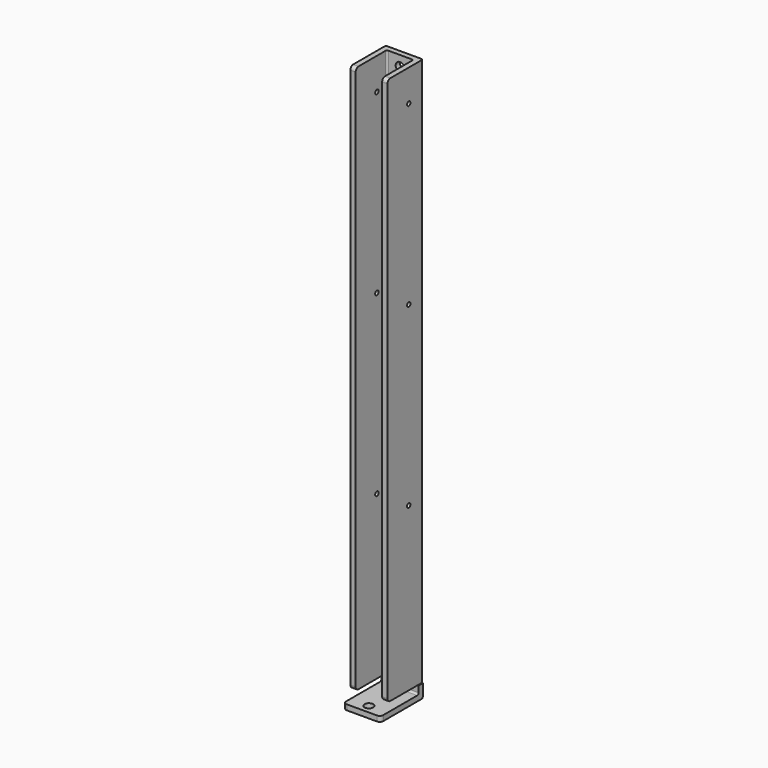
from build123d import *

# Parameters (mm, degrees)
F1_DEPTH  = 15
F2_W      = 3
F2_H      = 310
F3_DEPTH  = 25
F4_R      = 2.5
F5_DEPTH  = 3
F6_W      = 1
F6_H      = 0.5
F7_DEPTH  = 3
F8_R      = 1
F9_R      = 2.5
F9_R_2    = 1.2
F10_DEPTH = 3
F11_R     = 1.2
F12_DEPTH = 34.2
F13_DEPTH = 3
F14_DEPTH = 3
F15_R     = 2


with BuildPart() as f1:
    # F0 (on Right) → F1 (new body)
    with BuildSketch(Plane.YZ):
        Polygon((-7.5968508422, 3), (-7.5968508422, 0), (22.4031491578, 0), (22.4031491578, 318), (19.4031491578, 318), (19.4031491578, 3), align=None)
    extrude(amount=F1_DEPTH)

    # F2 (on face) → F3 (join)
    with BuildSketch(Plane(origin=(0, 22.4031491578, 0), x_dir=(-1, 0, 0), z_dir=(0, 1, 0))):
        with Locations((1.5, 163)):
            Rectangle(F2_W, F2_H)
        with Locations((-16.5, 163)):
            Rectangle(F2_W, F2_H)
    extrude(amount=-F3_DEPTH)

    # F4 (on face) → F5 (cut)
    with BuildSketch(Plane.XY.offset(3)):
        with Locations((7.5, -2.5968508422)):
            Circle(F4_R)
        with Locations((7.5, 12.4031491578)):
            Circle(F4_R)
    extrude(amount=-F5_DEPTH, mode=Mode.SUBTRACT)

    # F6 (on face) → F7 (cut)
    with BuildSketch(Plane.XZ.offset(-19.4031491578)):
        with Locations((0.5, 7.75)):
            Rectangle(F6_W, F6_H)
        with Locations((14.5, 7.75)):
            Rectangle(F6_W, F6_H)
    extrude(amount=-F7_DEPTH, mode=Mode.SUBTRACT)

    # F8
    f8_edges = [f1.edges().sort_by_distance(p)[0] for p in [
        (7.5, 19.403149, 3),
        (7.5, 22.403149, 0),
        (0, 19.403149, 163),
        (-3, 22.403149, 163),
        (18, 22.403149, 163),
        (15, 19.403149, 163),
    ]]
    fillet(f8_edges, radius=F8_R)

    # F9 (on face) → F10 (cut)
    with BuildSketch(Plane.XZ.offset(-19.4031491578)):
        with Locations((7.5, 312)):
            Circle(F9_R)
        with Locations((7.5, 100)):
            Circle(F9_R_2)
        with Locations((7.5, 200)):
            Circle(F9_R_2)
    extrude(amount=-F10_DEPTH, mode=Mode.SUBTRACT)

    # F11 (on face) → F12 (cut)
    with BuildSketch(Plane(origin=(-3, 0, 0), x_dir=(0, -1, 0), z_dir=(-1, 0, 0))):
        with Locations((-12.4031491578, 300)):
            Circle(F11_R)
        with Locations((-12.4031491578, 100)):
            Circle(F11_R)
        with Locations((-12.4031491578, 200)):
            Circle(F11_R)
    extrude(amount=-F12_DEPTH, mode=Mode.SUBTRACT)

    # F13 (add): a face of the model
    f13_faces = [f1.faces().sort_by_distance(p)[0] for p in [
        (0, 9.1577983799, 1.9953507779),
    ]]
    extrude(f13_faces, amount=F13_DEPTH)

    # F14 (add): a face of the model
    f14_faces = [f1.faces().sort_by_distance(p)[0] for p in [
        (15, 9.1577983799, 1.9953507779),
    ]]
    extrude(f14_faces, amount=F14_DEPTH)

    # F15
    f15_edges = [f1.edges().sort_by_distance(p)[0] for p in [
        (-1.5, -2.596851, 8),
        (16.5, -2.596851, 8),
        (-3, -7.596851, 1.5),
        (18, -7.596851, 1.5),
        (-1.5, -2.596851, 318),
        (16.5, -2.596851, 318),
    ]]
    fillet(f15_edges, radius=F15_R)


solid = f1.part
